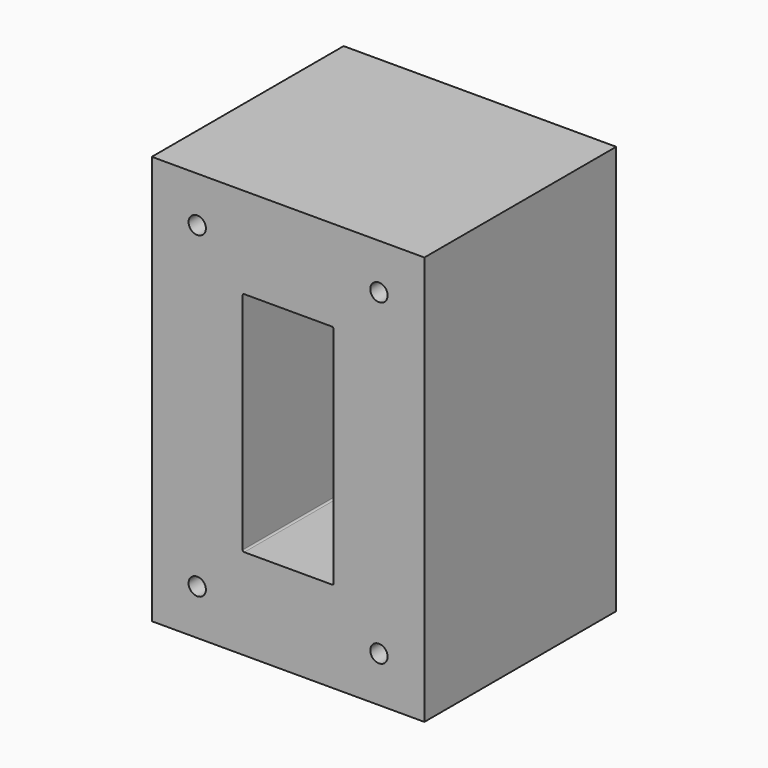
from build123d import *

# Parameters (mm, degrees)
F1_W     = 137.16
F1_H     = 205.74
F2_DEPTH = 120.65
F3_R     = 4.365625
F4_DEPTH = 120.65
F5_W     = 45.72
F5_H     = 114.3
F6_DEPTH = 120.65
F7_R     = 0.79375


# Not quite as in the source:
# - a variable given as a bare number and used for a length is read in inches; the dataset says mm whatever the document's units were


with BuildPart() as f2:
    # F1 (on Front) → F2 (new body)
    with BuildSketch(Plane.XZ):
        Rectangle(F1_W, F1_H)
    extrude(amount=-F2_DEPTH)

    # F3 (on face) → F4 (cut)
    with BuildSketch(Plane.XZ):
        with Locations((-45.72, 80.01)):
            Circle(F3_R)
        with Locations((45.72, 80.01)):
            Circle(F3_R)
        with Locations((-45.72, -80.01)):
            Circle(F3_R)
        with Locations((45.72, -80.01)):
            Circle(F3_R)
    extrude(amount=-F4_DEPTH, mode=Mode.SUBTRACT)

    # F5 (on face) → F6 (cut)
    with BuildSketch(Plane.XZ):
        Rectangle(F5_W, F5_H)
    extrude(amount=-F6_DEPTH, mode=Mode.SUBTRACT)

    # F7
    f7_edges = [f2.edges().sort_by_distance(p)[0] for p in [
        (-22.86, 60.325, 57.15),
        (22.86, 60.325, 57.15),
        (22.86, 60.325, -57.15),
        (-22.86, 60.325, -57.15),
    ]]
    fillet(f7_edges, radius=F7_R)


solid = f2.part
